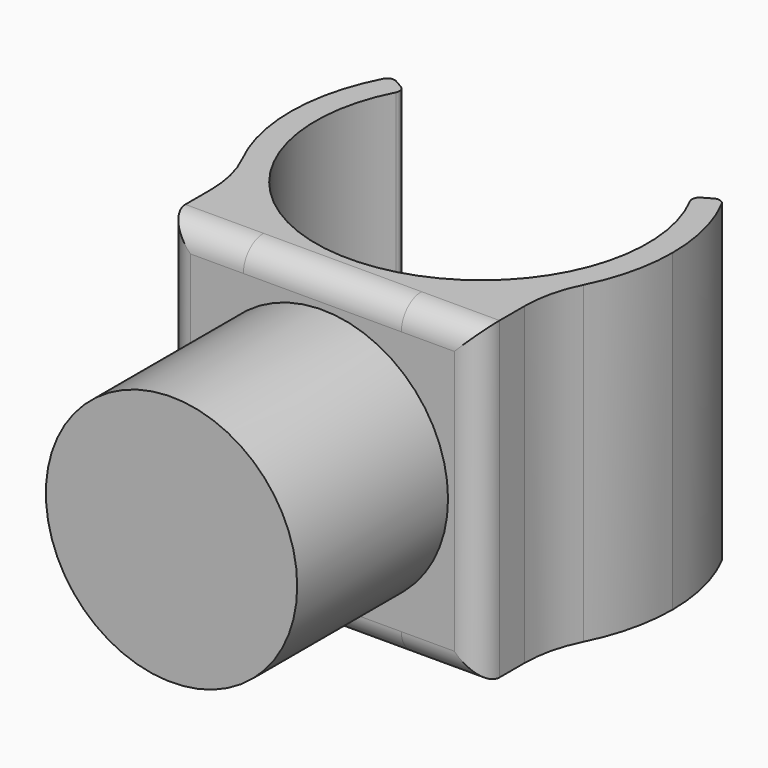
from build123d import *

# Parameters (mm, degrees)
F1_DEPTH    = 15.875
F2_DEPTH    = 15.875
F3_R        = 12.7
F4_DEPTH    = 19.05
F5_R        = 2.54
F6_T1_DEPTH = 31.75
F7_R        = 0.762


# Not quite as in the source:
# - a fillet or chamfer that OpenCascade refuses, or shapes differently, is made with other operations: its cross-section is extruded or revolved along the edge and cut away or added


with BuildPart() as f1:
    # F0 (on Top) → F1 (new body, symmetric)
    with BuildSketch(Plane.XY):
        with BuildLine():
            ThreePointArc((15.875, -10.9831139027), (18.4268203443, -5.7529738397), (19.304, 0))
            ThreePointArc((19.304, 0), (18.6462321507, 4.9962428467), (16.7177543947, 9.652))
            Line((16.7177543947, 9.652), (14.518049869, 8.382))
            ThreePointArc((14.518049869, 8.382), (16.1927805519, 4.3388424721), (16.764, 0))
            ThreePointArc((16.764, 0), (-4.3388424721, -16.1927805519), (-14.518049869, 8.382))
            Line((-14.518049869, 8.382), (-16.7177543947, 9.652))
            ThreePointArc((-16.7177543947, 9.652), (-19.2879208626, -0.7877339639), (-15.875, -10.9831139027))
            ThreePointArc((-15.875, -10.9831139027), (0, -19.304), (15.875, -10.9831139027))
        make_face()
    extrude(amount=F1_DEPTH, both=True)

    # F0 (on Top) → F2 (join, symmetric)
    with BuildSketch(Plane.XY):
        with BuildLine():
            Line((15.875, -20.1168), (15.875, -10.9831139027))
            ThreePointArc((15.875, -10.9831139027), (0, -19.304), (-15.875, -10.9831139027))
            Line((-15.875, -10.9831139027), (-15.875, -20.1168))
            Line((-15.875, -20.1168), (15.875, -20.1168))
        make_face()
    extrude(amount=F2_DEPTH, both=True)

    # F3 (on face) → F4 (join)
    with BuildSketch(Plane.XZ.offset(20.1168)):
        Circle(F3_R)
    extrude(amount=F4_DEPTH)

    # F5
    f5_edges = [f1.edges().sort_by_distance(p)[0] for p in [
        (-15.875, -20.1168, 0),
        (15.875, -20.1168, 0),
        (0, -20.1168, 15.875),
        (0, -20.1168, -15.875),
    ]]
    fillet(f5_edges, radius=F5_R)

    # F6: fillet of radius 12.7 on 2 edges, made by hand

    # F6_s2 → F6_t1 (join)
    with BuildSketch(Plane.XY.offset(-15.875)):
        with BuildLine():
            ThreePointArc((-15.875, -14.4126816034), (-16.2198608148, -11.4732027866), (-17.2357142857, -8.6933635068))
            ThreePointArc((-17.2357142857, -8.6933635068), (-16.594896485, -9.8617354788), (-15.875, -10.9831139027))
            Line((-15.875, -10.9831139027), (-15.875, -14.4126816034))
        make_face()
        with BuildLine():
            ThreePointArc((15.875, -14.4126816034), (16.2198608148, -11.4732027866), (17.2357142857, -8.6933635068))
            ThreePointArc((17.2357142857, -8.6933635068), (16.594896485, -9.8617354788), (15.875, -10.9831139027))
            Line((15.875, -10.9831139027), (15.875, -14.4126816034))
        make_face()
    extrude(amount=F6_T1_DEPTH)

    # F7
    f7_edges = [f1.edges().sort_by_distance(p)[0] for p in [
        (-16.717754, 9.652, 0),
        (-14.51805, 8.382, 0),
        (16.717754, 9.652, 0),
        (14.51805, 8.382, 0),
    ]]
    fillet(f7_edges, radius=F7_R)


solid = f1.part
